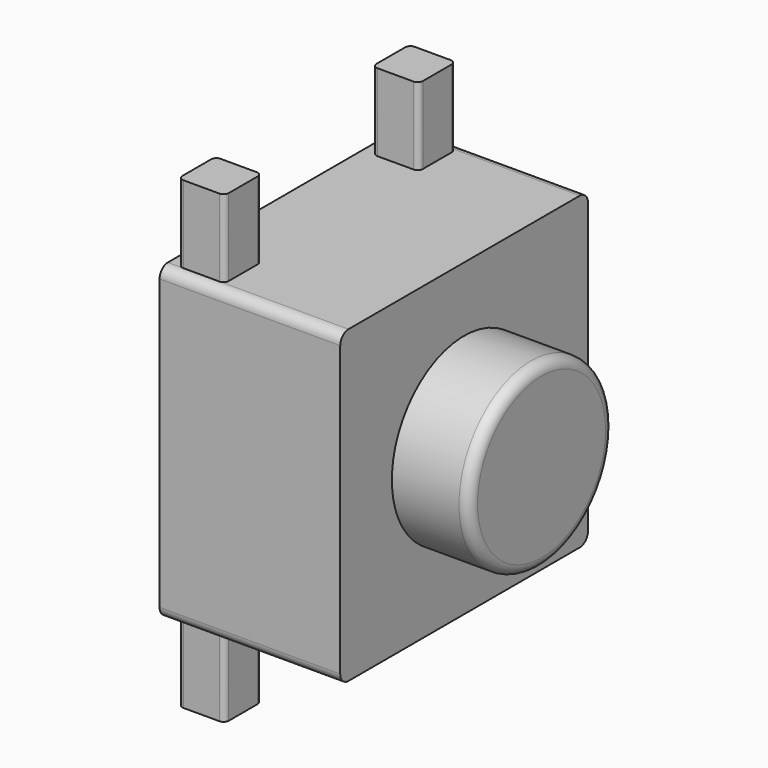
from build123d import *

# Parameters (mm, degrees)
F0_W     = 6
F0_H     = 6
F1_DEPTH = 1.75
F2_R     = 1.75
F3_DEPTH = 1.5
F4_R     = 0.2
F6_DEPTH = 1.5


# Not quite as in the source:
# - a pattern or mirror of a feature is missing from the dataset's text; its kind, count and spacing are read off the source's solid


with BuildPart() as f1:
    # F0 (on Right) → F1 (new body, symmetric)
    with BuildSketch(Plane.YZ):
        Rectangle(F0_W, F0_H)
    extrude(amount=F1_DEPTH, both=True)

    # F2 (on face) → F3 (join)
    with BuildSketch(Plane.YZ.offset(1.75)):
        Circle(F2_R)
    extrude(amount=F3_DEPTH)

    # F4
    f4_edges = [f1.edges().sort_by_distance(p)[0] for p in [
        (3.25, -1.75, 0),
        (0, -3, 3),
        (0, 3, 3),
        (0, 3, -3),
        (0, -3, -3),
    ]]
    fillet(f4_edges, radius=F4_R)

    # F5 (on face) → F6 (join)
    with BuildSketch(Plane.XY.offset(3)):
        with BuildLine():
            ThreePointArc((-1.55, -2.7), (-1.5207106781, -2.7707106781), (-1.45, -2.8))
            Line((-1.45, -2.8), (-0.75, -2.8))
            ThreePointArc((-0.75, -2.8), (-0.6792893219, -2.7707106781), (-0.65, -2.7))
            Line((-0.65, -2.7), (-0.65, -2))
            ThreePointArc((-0.65, -2), (-0.6792893219, -1.9292893219), (-0.75, -1.9))
            Line((-0.75, -1.9), (-1.45, -1.9))
            ThreePointArc((-1.45, -1.9), (-1.5207106781, -1.9292893219), (-1.55, -2))
            Line((-1.55, -2), (-1.55, -2.7))
        make_face()
        with BuildLine():
            ThreePointArc((-0.65, 2.7), (-0.6792893219, 2.7707106781), (-0.75, 2.8))
            Line((-0.75, 2.8), (-1.45, 2.8))
            ThreePointArc((-1.45, 2.8), (-1.5207106781, 2.7707106781), (-1.55, 2.7))
            Line((-1.55, 2.7), (-1.55, 2))
            ThreePointArc((-1.55, 2), (-1.5207106781, 1.9292893219), (-1.45, 1.9))
            Line((-1.45, 1.9), (-0.75, 1.9))
            ThreePointArc((-0.75, 1.9), (-0.6792893219, 1.9292893219), (-0.65, 2))
            Line((-0.65, 2), (-0.65, 2.7))
        make_face()
    f6 = extrude(amount=F6_DEPTH)

    # F6_copies: F6 across plane
    add(f6.mirror(Plane(origin=(0, 0, 0), x_dir=(-1, 0, 0), z_dir=(0, 0, -1))))


solid = f1.part
